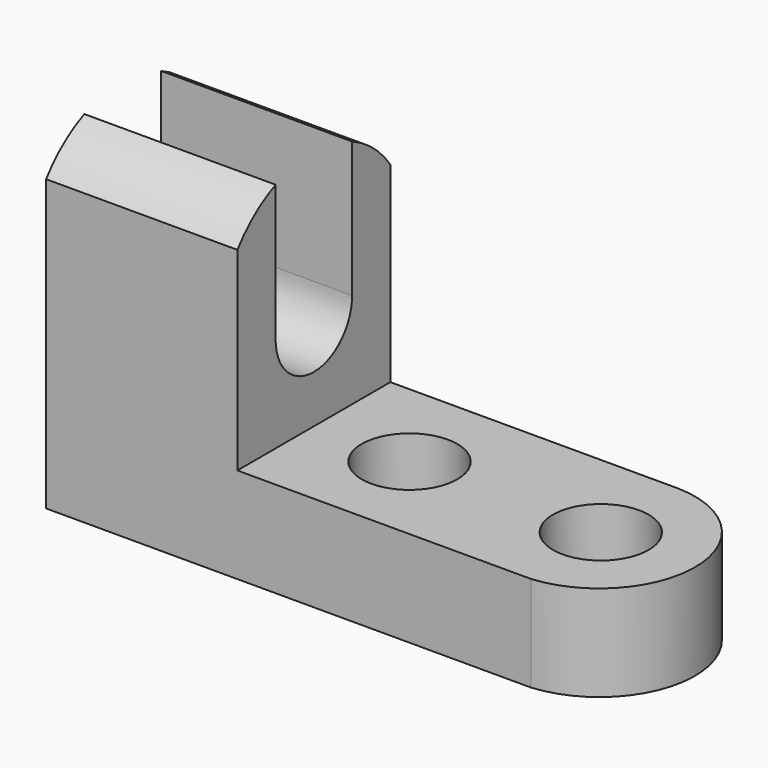
from build123d import *

# Parameters (mm, degrees)
F1_DEPTH = 25.4
F2_R     = 6.35
F3_DEPTH = 25.4
F5_DEPTH = 76.201
F7_DEPTH = 25.401
F9_DEPTH = 12.701


# Not quite as in the source:
# - ends of sketch curves that miss each other by under 0.0002 mm in the source are joined


with BuildPart() as f1:
    # F0 (on Front) → F1 (new body)
    with BuildSketch(Plane.XZ):
        Polygon((-50.8, 44.45), (-76.2, 44.45), (-76.2, 0), (0, 0), (0, 12.7), (-50.8, 12.7), align=None)
    extrude(amount=F1_DEPTH)

    # F2 (on face) → F3 (cut)
    with BuildSketch(Plane.XY.offset(12.7)):
        with Locations((-38.1, -12.7)):
            Circle(F2_R)
        with Locations((-12.7, -12.7)):
            Circle(F2_R)
    extrude(amount=-F3_DEPTH, mode=Mode.SUBTRACT)

    # F4 (on Right) → F5 (cut, through all)
    with BuildSketch(Plane.YZ):
        with BuildLine():
            ThreePointArc((-19.05, 25.4), (-12.7, 19.05), (-6.35, 25.4))
            ThreePointArc((-6.35, 25.4), (-12.7, 31.75), (-19.05, 25.4))
        make_face()
        with BuildLine():
            ThreePointArc((-19.05, 25.4), (-12.7, 31.75), (-6.35, 25.4))
            Line((-6.35, 25.4), (-6.3499049408, 44.4847454087))
            Line((-6.3499049408, 44.4847454087), (-19.05, 44.5389002562))
            Line((-19.05, 44.5389002562), (-19.05, 25.4))
        make_face()
    extrude(amount=-F5_DEPTH, mode=Mode.SUBTRACT)

    # F6 (on face) → F7 (cut, through all)
    with BuildSketch(Plane.YZ.offset(-50.8)):
        with BuildLine():
            ThreePointArc((-25.4, 38.4937003255), (-22.5556194367, 41.4256632835), (-19.05, 43.5226945042))
            Line((-19.05, 43.5226945042), (-19.05, 44.45))
            Line((-19.05, 44.45), (-25.4, 44.45))
            Line((-25.4, 44.45), (-25.4, 38.4937003255))
        make_face()
        with BuildLine():
            ThreePointArc((-6.3499103, 43.4087842374), (-2.8217014128, 41.1990275697), (0, 38.1380990148))
            Line((0, 38.1380990148), (0, 44.45))
            Line((0, 44.45), (-6.3499051138, 44.45))
            Line((-6.3499051138, 44.45), (-6.3499103, 43.4087842374))
        make_face()
    extrude(amount=-F7_DEPTH, mode=Mode.SUBTRACT)

    # F8 (on face) → F9 (cut, through all)
    with BuildSketch(Plane.XY.offset(12.7)):
        with BuildLine():
            ThreePointArc((-12.5391965152, 0), (-0.172750427, -12.3617250524), (-11.8236998096, -25.4))
            Line((-11.8236998096, -25.4), (0, -25.4))
            Line((0, -25.4), (0, 0))
            Line((0, 0), (-12.5391965152, 0))
        make_face()
    extrude(amount=-F9_DEPTH, mode=Mode.SUBTRACT)


solid = f1.part
